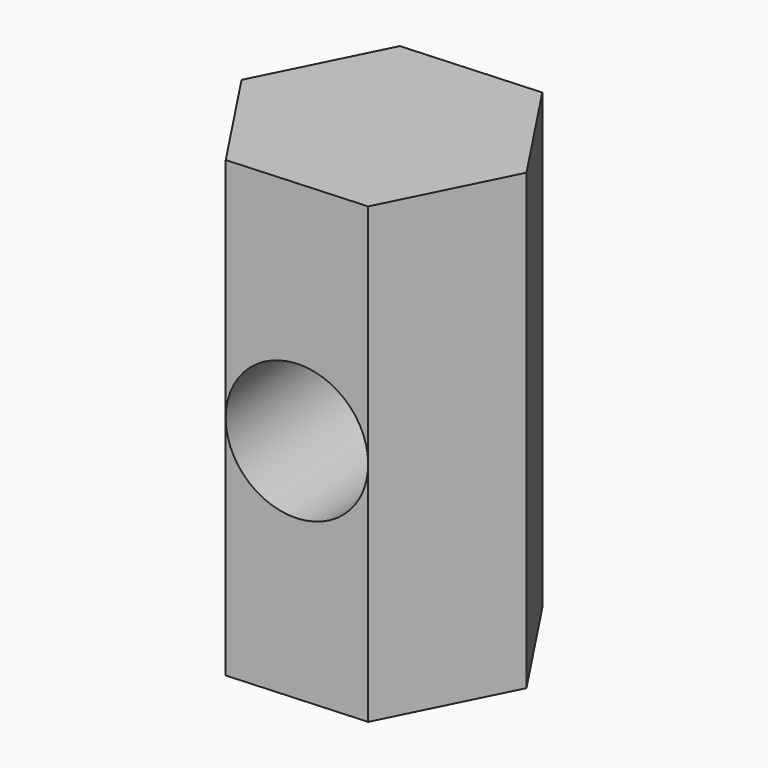
from build123d import *

# Parameters (mm, degrees)
F1_DEPTH = 10
F3_DEPTH = 5.1961524227


with BuildPart() as f1:
    # F0 (on Top) → F1 (new body)
    with BuildSketch(Plane.XY):
        Polygon((-1.3409011788, -2.6836512495), (1.6536595675, -2.5030801095), (2.9945607463, 0.18057114), (1.3409011788, 2.6836512495), (-1.6536595675, 2.5030801095), (-2.9945607463, -0.18057114), align=None)
    extrude(amount=F1_DEPTH)

    # F2 (on face) → F3 (cut, through all)
    with BuildSketch(Plane(origin=(0.1563791944, -2.5933656795, 0), x_dir=(0.9981869154, 0.06019038, 0), z_dir=(0.06019038, -0.9981869154, 0))):
        with BuildLine():
            ThreePointArc((-1.5, 5), (0, 3.5), (1.5, 5))
            ThreePointArc((1.5, 5), (0, 6.5), (-1.5, 5))
        make_face()
    extrude(amount=-F3_DEPTH, mode=Mode.SUBTRACT)


solid = f1.part
